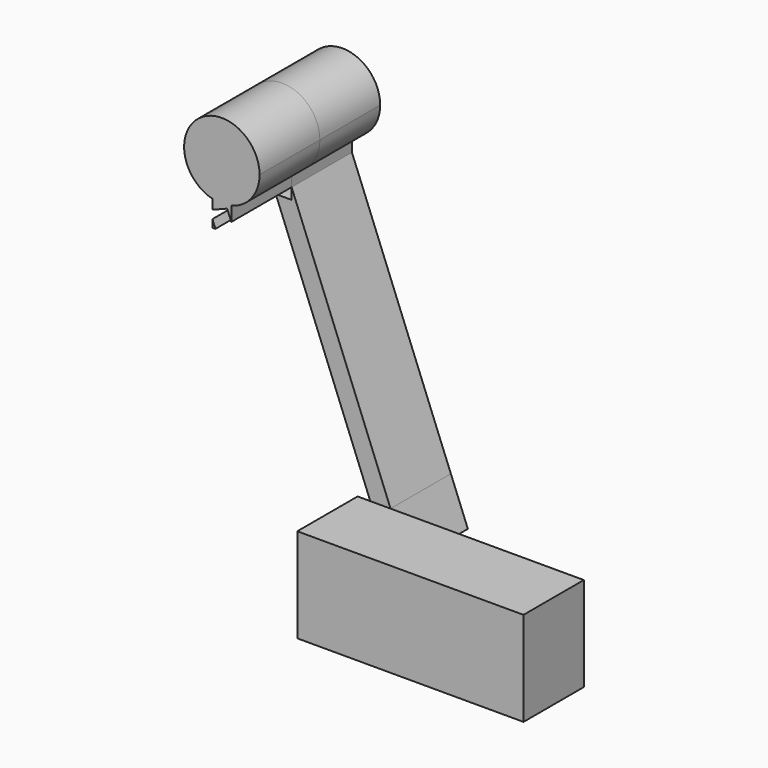
from build123d import *

# Parameters (mm, degrees)
F1_DEPTH = 25.4
F2_DEPTH = 25.4
F0_W     = 76.2
F0_H     = 6.35
F3_DEPTH = 25.4


# Not quite as in the source:
# - a feature names something its author has since deleted; it is built from what else it names


with BuildPart() as f1:
    # F0 (on Front) → F1 (new body)
    with BuildSketch(Plane.XZ):
        with BuildLine():
            ThreePointArc((3.175, -12.2967221242), (10.040231571, -7.7771299333), (12.7, 0))
            ThreePointArc((12.7, 0), (-7.7771299333, 10.040231571), (-3.175, -12.2967221242))
            Line((-3.175, -12.2967221242), (-3.175, 3.175))
            Line((-3.175, 3.175), (3.175, 3.175))
            Line((3.175, 3.175), (3.175, -12.2967221242))
        make_face()
        with BuildLine():
            Line((-3.175, 3.175), (-3.175, -12.2967221242))
            ThreePointArc((-3.175, -12.2967221242), (0, -12.7), (3.175, -12.2967221242))
            Line((3.175, -12.2967221242), (3.175, 3.175))
            Line((3.175, 3.175), (-3.175, 3.175))
        make_face()
        with BuildLine():
            ThreePointArc((3.175, -12.2967221242), (0, -12.7), (-3.175, -12.2967221242))
            Line((-3.175, -12.2967221242), (-3.175, -15.5686634239))
            Line((-3.175, -15.5686634239), (1.7882290969, -13.6105246429))
            Line((1.7882290969, -13.6105246429), (3.175, -17.1255266252))
            Line((3.175, -17.1255266252), (3.175, -12.2967221242))
        make_face()
    extrude(amount=F1_DEPTH)


with BuildPart() as f1b:
    # F0 (on Front) → F1, piece 2 (new body)
    with BuildSketch(Plane.XZ):
        Polygon((-2.1605365761, -20.9042), (-3.175, -18.3328733748), (-3.175, -20.9042), align=None)
    extrude(amount=F1_DEPTH)


with BuildPart() as f2:
    # F0 (on Front) → F2 (new body)
    with BuildSketch(Plane.XZ):
        with BuildLine():
            ThreePointArc((3.175, -12.2967221242), (10.040231571, -7.7771299333), (12.7, 0))
            ThreePointArc((12.7, 0), (-7.7771299333, 10.040231571), (-3.175, -12.2967221242))
            Line((-3.175, -12.2967221242), (-3.175, 3.175))
            Line((-3.175, 3.175), (3.175, 3.175))
            Line((3.175, 3.175), (3.175, -12.2967221242))
        make_face()
        with BuildLine():
            Line((-3.175, 3.175), (-3.175, -12.2967221242))
            ThreePointArc((-3.175, -12.2967221242), (0, -12.7), (3.175, -12.2967221242))
            Line((3.175, -12.2967221242), (3.175, 3.175))
            Line((3.175, 3.175), (-3.175, 3.175))
        make_face()
        with BuildLine():
            ThreePointArc((3.175, -12.2967221242), (0, -12.7), (-3.175, -12.2967221242))
            Line((-3.175, -12.2967221242), (-3.175, -15.5686634239))
            Line((-3.175, -15.5686634239), (1.7882290969, -13.6105246429))
            Line((1.7882290969, -13.6105246429), (3.175, -17.1255266252))
            Line((3.175, -17.1255266252), (3.175, -12.2967221242))
        make_face()
    extrude(amount=-F2_DEPTH)


with BuildPart() as f2b:
    # F0 (on Front) → F2, piece 2 (new body)
    with BuildSketch(Plane.XZ):
        Polygon((-3.175, -18.3328733748), (-3.175, -15.5686634239), (-4.1186753571, -15.9409709031), align=None)
    extrude(amount=-F2_DEPTH)


with BuildPart() as f2c:
    # F0 (on Front) → F2, piece 3 (new body)
    with BuildSketch(Plane.XZ):
        Polygon((36.5026459921, -101.6), (3.175, -17.1255266252), (3.175, -20.9042), (-2.1605365761, -20.9042), (29.6763124508, -101.6), align=None)
        Polygon((42.2186753571, -116.0882290969), (36.5026459921, -101.6), (29.6763124508, -101.6), (36.3117709031, -118.4186753571), align=None)
    extrude(amount=-F2_DEPTH)


with BuildPart() as f3:
    # F0 (on Front) → F3 (new body)
    with BuildSketch(Plane.XZ):
        Polygon((101.6, -101.6), (36.5026459921, -101.6), (42.2186753571, -116.0882290969), (36.3117709031, -118.4186753571), (29.6763124508, -101.6), (25.4, -101.6), (25.4, -127), (101.6, -127), align=None)
        Polygon((42.2186753571, -116.0882290969), (36.5026459921, -101.6), (29.6763124508, -101.6), (36.3117709031, -118.4186753571), align=None)
        with Locations((63.5, -130.175)):
            Rectangle(F0_W, F0_H)
    extrude(amount=F3_DEPTH)


solid = Compound([f1.part, f1b.part, f2.part, f2b.part, f2c.part, f3.part])
